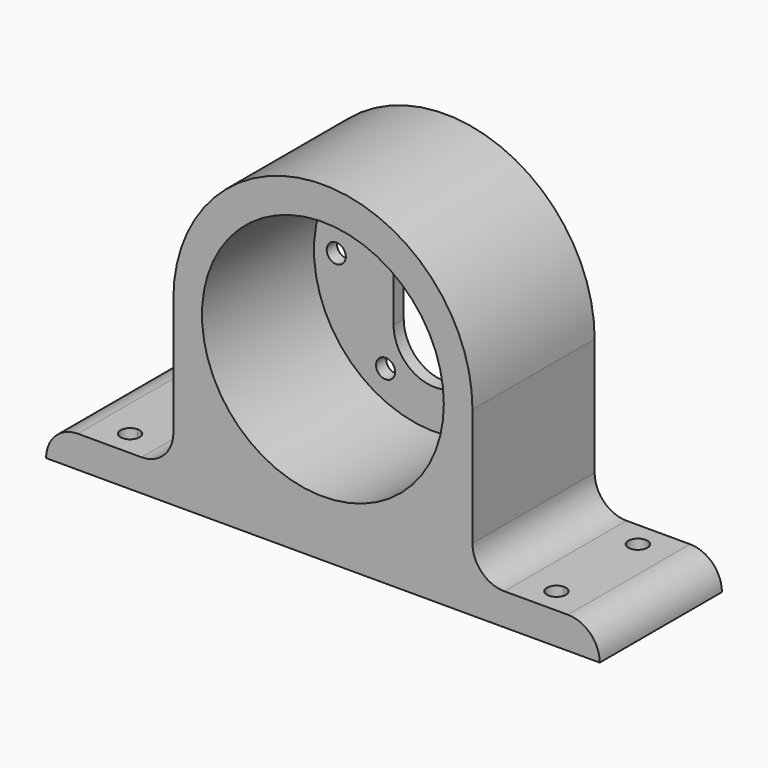
from build123d import *

# Parameters (mm, degrees)
F1_DEPTH  = 2
F2_R      = 1.5
F3_DEPTH  = 5
F4_R      = 19
F5_DEPTH  = 24
F6_W      = 47
F6_H      = 24
F7_DEPTH  = 5
F8_W      = 24
F8_H      = 5
F9_DEPTH  = 20
F11_DEPTH = 25
F12_W     = 24
F12_H     = 5
F13_DEPTH = 20
F15_DEPTH = 25
F16_R     = 4.99999


# Not quite as in the source:
# - a fillet or chamfer is up to 0.001 mm smaller than in the source, because OpenCascade refuses the exact size


with BuildPart() as f1:
    # F0 (on Front) → F1 (new body)
    with BuildSketch(Plane.XZ):
        with BuildLine():
            Line((-23.5, -23.5), (0, -23.5))
            Line((0, -23.5), (23.5, -23.5))
            Line((23.5, -23.5), (23.5, 0))
            ThreePointArc((23.5, 0), (0, 23.5), (-23.5, 0))
            Line((-23.5, 0), (-23.5, -23.5))
        make_face()
    extrude(amount=F1_DEPTH)

    # F2 (on face) → F3 (cut)
    with BuildSketch(Plane.XZ.offset(2)):
        with Locations((15.5, 0)):
            Circle(F2_R)
        with Locations((7.75, 13.4233937587)):
            Circle(F2_R)
        with Locations((-7.75, 13.4233937587)):
            Circle(F2_R)
        with Locations((-15.5, 0)):
            Circle(F2_R)
        with Locations((-7.75, -13.4233937587)):
            Circle(F2_R)
        with Locations((7.75, -13.4233937587)):
            Circle(F2_R)
        with BuildLine():
            Line((6.5, -7), (6.5, 7))
            ThreePointArc((6.5, 7), (0, 13.5), (-6.5, 7))
            Line((-6.5, 7), (-6.5, -7))
            ThreePointArc((-6.5, -7), (0, -13.5), (6.5, -7))
        make_face()
    extrude(amount=-F3_DEPTH, mode=Mode.SUBTRACT)

    # F4 (on Front) → F5 (join)
    with BuildSketch(Plane.XZ):
        with BuildLine():
            ThreePointArc((23.5, 0), (0, 23.5), (-23.5, 0))
            Line((-23.5, 0), (-23.5, -23.5))
            Line((-23.5, -23.5), (23.5, -23.5))
            Line((23.5, -23.5), (23.5, 0))
        make_face()
        with Locations((0, -0.6784388353)):
            Circle(F4_R, mode=Mode.SUBTRACT)
    extrude(amount=F5_DEPTH)

    # F6 (on face) → F7 (join)
    with BuildSketch(Plane(origin=(0, 0, -23.5), x_dir=(1, 0, 0), z_dir=(0, 0, -1))):
        with Locations((0, 12)):
            Rectangle(F6_W, F6_H)
    extrude(amount=F7_DEPTH)

    # F8 (on face) → F9 (join)
    with BuildSketch(Plane(origin=(-23.5, 0, 0), x_dir=(0, -1, 0), z_dir=(-1, 0, 0))):
        with Locations((12, -26)):
            Rectangle(F8_W, F8_H)
    extrude(amount=F9_DEPTH)

    # F10 (on face) → F11 (cut)
    with BuildSketch(Plane.XY.offset(-23.5)):
        with BuildLine():
            ThreePointArc((-32, -4), (-34.5606601718, -2.9393398282), (-33.5, -5.5))
            ThreePointArc((-33.5, -5.5), (-32.4393398282, -5.0606601718), (-32, -4))
        make_face()
        with BuildLine():
            ThreePointArc((-32, -20), (-32.4393398282, -18.9393398282), (-33.5, -18.5))
            ThreePointArc((-33.5, -18.5), (-34.5606601718, -21.0606601718), (-32, -20))
        make_face()
    extrude(amount=-F11_DEPTH, mode=Mode.SUBTRACT)

    # F12 (on face) → F13 (join)
    with BuildSketch(Plane.YZ.offset(23.5)):
        with Locations((-12, -26)):
            Rectangle(F12_W, F12_H)
    extrude(amount=F13_DEPTH)

    # F14 (on face) → F15 (cut)
    with BuildSketch(Plane.XY.offset(-23.5)):
        with BuildLine():
            ThreePointArc((35, -4), (32.4393398282, -2.9393398282), (33.5, -5.5))
            ThreePointArc((33.5, -5.5), (34.5606601718, -5.0606601718), (35, -4))
        make_face()
        with BuildLine():
            ThreePointArc((35, -20), (34.5606601718, -18.9393398282), (33.5, -18.5))
            ThreePointArc((33.5, -18.5), (32.4393398282, -21.0606601718), (35, -20))
        make_face()
    extrude(amount=-F15_DEPTH, mode=Mode.SUBTRACT)

    # F16 (radius 5 in the source; OpenCascade refuses exactly that, so slightly less here)
    f16_edges = [f1.edges().sort_by_distance(p)[0] for p in [
        (23.5, -12, -23.5),
        (43.5, -12, -23.5),
        (-23.5, -12, -23.5),
        (-43.5, -12, -23.5),
    ]]
    fillet(f16_edges, radius=F16_R)


solid = f1.part
